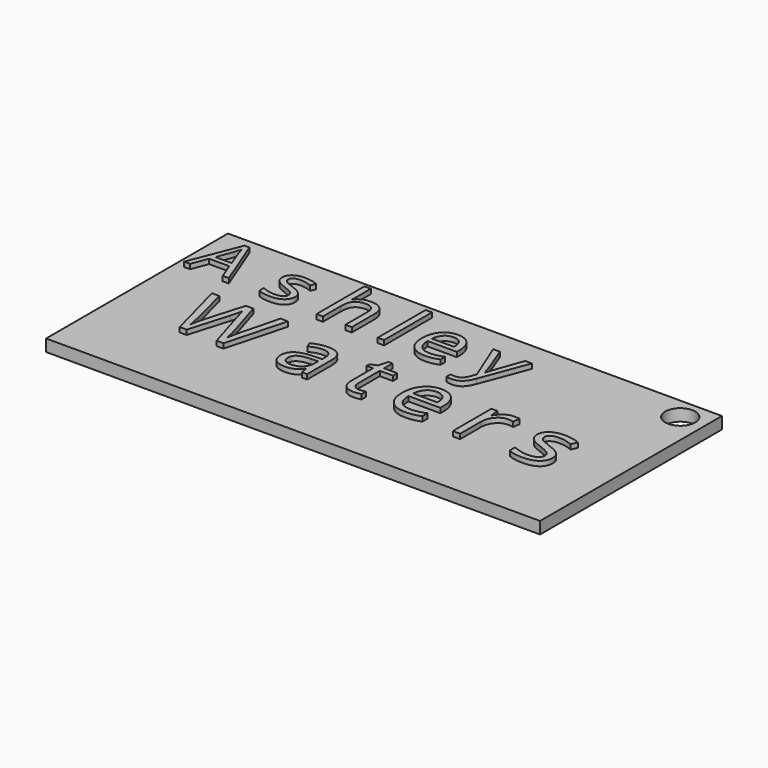
from build123d import *

# Parameters (mm, degrees)
F0_W           = 105.0491034985
F0_H           = 48.3513679355
F1_DEPTH       = 2.54
F3_D           = 6.35
F2_TEXT_SIZE   = 15.0004443916
F2_TEXT_SIZE_2 = 15.9892098357
F2_TEXT_SIZE_3 = 16.7886687753
F2_TEXT_SIZE_4 = 16.3889399523
F2_TEXT_SIZE_5 = 17.9878597717
F2_TEXT_SIZE_6 = 18.3875898882
F2_TEXT_SIZE_7 = 19.1870501213
F4_DEPTH       = 1.016


# Not quite as in the source:
# - Text() gives the source's letters only with a copy of the font that has no kerning and outlines rounded to 1/6400 em; it was checked with that copy


with BuildPart() as f1:
    # F0 (on Top) → F1 (new body)
    with BuildSketch(Plane.XY):
        with Locations((0.8634179831, 1.8707374111)):
            Rectangle(F0_W, F0_H)
    extrude(amount=F1_DEPTH)

    # F3 (through all)
    with Locations(Plane(origin=(0, 0, 0), x_dir=(1, 0, 0), z_dir=(0, 0, -1))):
        with Locations((48.2074655592, -21.4415285736)):
            Hole(F3_D / 2)

    # F2 (on face) → F4 (join)
    with BuildSketch(Plane.XY.offset(2.54)):
        with Locations((-49.8022324642, 12.0802379625)):
            Text('A', F2_TEXT_SIZE, font='Open Sans', text_align=(TextAlign.LEFT, TextAlign.BOTTOM))
        with Locations((-34.3927890062, 11.3683268428)):
            Text('s', F2_TEXT_SIZE_2, font='Open Sans', text_align=(TextAlign.LEFT, TextAlign.BOTTOM))
        with Locations((-22.3049465567, 11.0805211589)):
            Text('h', F2_TEXT_SIZE_3, font='Open Sans', text_align=(TextAlign.LEFT, TextAlign.BOTTOM))
        with Locations((-9.0658813715, 10.7927164063)):
            Text('l', F2_TEXT_SIZE_3, font='Open Sans', text_align=(TextAlign.LEFT, TextAlign.BOTTOM))
        with Locations((-2.7341546956, 10.7927164063)):
            Text('e', F2_TEXT_SIZE_3, font='Open Sans', text_align=(TextAlign.LEFT, TextAlign.BOTTOM))
        with Locations((9.9292984232, 10.7927164063)):
            Text('y', F2_TEXT_SIZE_4, font='Open Sans', text_align=(TextAlign.LEFT, TextAlign.BOTTOM))
        with Locations((-39.3370786816, -6.7634354346)):
            Text('W', F2_TEXT_SIZE_5, font='Open Sans', text_align=(TextAlign.LEFT, TextAlign.BOTTOM))
        with Locations((-17.1244423836, -6.7634354346)):
            Text('a', F2_TEXT_SIZE_5, font='Open Sans', text_align=(TextAlign.LEFT, TextAlign.BOTTOM))
        with Locations((-3.0219603796, -6.7634354346)):
            Text('t', F2_TEXT_SIZE_5, font='Open Sans', text_align=(TextAlign.LEFT, TextAlign.BOTTOM))
        with Locations((6.8957207847, -7.0512411185)):
            Text('e', F2_TEXT_SIZE_6, font='Open Sans', text_align=(TextAlign.LEFT, TextAlign.BOTTOM))
        with Locations((21.4415285736, -7.6268524863)):
            Text('r', F2_TEXT_SIZE_7, font='Open Sans', text_align=(TextAlign.LEFT, TextAlign.BOTTOM))
        with Locations((33.8171757758, -7.6268524863)):
            Text('s', F2_TEXT_SIZE_7, font='Open Sans', text_align=(TextAlign.LEFT, TextAlign.BOTTOM))
    extrude(amount=F4_DEPTH)


solid = f1.part
